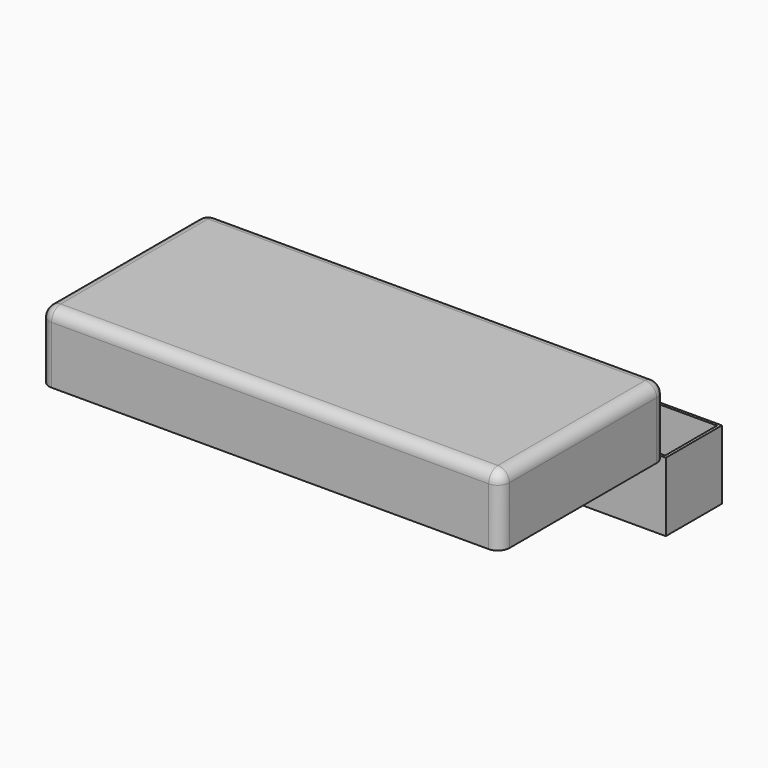
from build123d import *

# Parameters (mm, degrees)
F0_W     = 2000
F0_H     = 900
F1_DEPTH = 300
F2_R     = 50
F3_T     = 50
F5_DEPTH = 300
F6_T     = -12


# Not quite as in the source:
# - a shell that OpenCascade refuses in one call is made with other operations: the cavity is built on its own and cut out


with BuildPart() as f1:
    # F0 (on Top) → F1 (new body)
    with BuildSketch(Plane.XY):
        with Locations((-167.8199538224, -450)):
            Rectangle(F0_W, F0_H)
    extrude(amount=F1_DEPTH)

    # F2
    f2_edges = [f1.edges().sort_by_distance(p)[0] for p in [
        (-167.819954, -900, 300),
        (832.180046, -450, 300),
        (-167.819954, 0, 300),
        (-1167.819954, -450, 300),
        (-1167.819954, -900, 150),
        (832.180046, -900, 150),
        (832.180046, 0, 150),
        (-1167.819954, 0, 150),
    ]]
    fillet(f2_edges, radius=F2_R)

    # F3: shell of thickness 50, made by hand


with BuildPart() as f3_core1:
    # F3_t2: copy of F1
    add(f1.part)

    # the walls: a layer under each face that stays
    f3_faces = [f3_core1.faces().sort_by_distance(p)[0] for p in [
        (-167.8199538224, 0, 125),
        (832.1800461776, -450, 125),
        (-1167.8199538224, -450, 125),
        (-167.8199538224, -900, 125),
        (-167.8199538224, -450, 300),
    ]]
    thicken(f3_faces, amount=-F3_T, mode=Mode.SUBTRACT)


with BuildPart() as f1_1:
    add(f1.part)

    # what is left inside the walls is the cavity
    f3_cavity = [f3_core1.part.solids().sort_by_distance(p)[0] for p in [
        (-167.819954, -583.333333, 0.5),
    ]]
    add(f3_cavity, mode=Mode.SUBTRACT)


with BuildPart() as f5:
    # F4 (on face) → F5 (new body)
    with BuildSketch(Plane(origin=(0, 0, 0), x_dir=(1, 0, 0), z_dir=(0, 0, -1))):
        Polygon((782.1800461776, 0), (-1117.8199538224, 0), (-1167.8199538224, 0), (-1167.8199538224, -305), (832.1800461776, -305), (832.1800461776, 0), align=None)
    extrude(amount=F5_DEPTH)

    # F6
    f6_openings = [f5.faces().sort_by_distance(p)[0] for p in [
        (-167.819954, 152.5, 0),
    ]]
    offset(amount=F6_T, openings=f6_openings)


solid = Compound([f1_1.part, f5.part])
